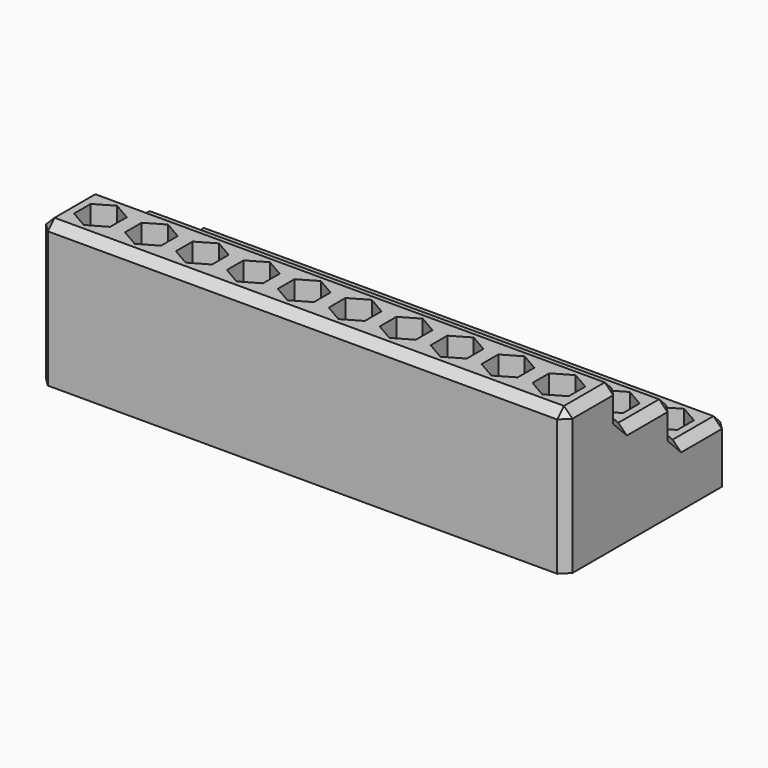
from build123d import *

# Parameters (mm, degrees)
F2_W     = 62
F2_H     = 8
F3_DEPTH = 17
F4_DEPTH = 12
F5_DEPTH = 7
F6_DEPTH = 8
F7_DEPTH = 13
F8_DEPTH = 18
F9_SIZE  = 1


with BuildPart() as f3:
    # F2 (on offset) → F3 (new body)
    with BuildSketch(Plane.XY.offset(-20)):
        with Locations((31, 4)):
            Rectangle(F2_W, F2_H)
    extrude(amount=F3_DEPTH)

    # F2 (on offset) → F4 (join)
    with BuildSketch(Plane.XY.offset(-20)):
        with Locations((31, 12)):
            Rectangle(F2_W, F2_H)
    extrude(amount=F4_DEPTH)

    # F2 (on offset) → F5 (join)
    with BuildSketch(Plane.XY.offset(-20)):
        with Locations((31, 20)):
            Rectangle(F2_W, F2_H)
    extrude(amount=F5_DEPTH)

    # F0 (on Top) → F6 (cut)
    with BuildSketch(Plane.XY):
        Polygon((58, 6.4537386441), (55.875, 5.226869322), (55.875, 2.773130678), (58, 1.5462613559), (60.125, 2.773130678), (60.125, 5.226869322), align=None)
        Polygon((52, 6.4537386441), (49.875, 5.226869322), (49.875, 2.773130678), (52, 1.5462613559), (54.125, 2.773130678), (54.125, 5.226869322), align=None)
        Polygon((46, 6.4537386441), (43.875, 5.226869322), (43.875, 2.773130678), (46, 1.5462613559), (48.125, 2.773130678), (48.125, 5.226869322), align=None)
        Polygon((40, 6.4537386441), (37.875, 5.226869322), (37.875, 2.773130678), (40, 1.5462613559), (42.125, 2.773130678), (42.125, 5.226869322), align=None)
        Polygon((34, 6.4537386441), (31.875, 5.226869322), (31.875, 2.773130678), (34, 1.5462613559), (36.125, 2.773130678), (36.125, 5.226869322), align=None)
        Polygon((28, 6.4537386441), (25.875, 5.226869322), (25.875, 2.773130678), (28, 1.5462613559), (30.125, 2.773130678), (30.125, 5.226869322), align=None)
        Polygon((22, 6.4537386441), (19.875, 5.226869322), (19.875, 2.773130678), (22, 1.5462613559), (24.125, 2.773130678), (24.125, 5.226869322), align=None)
        Polygon((16, 6.4537386441), (13.875, 5.226869322), (13.875, 2.773130678), (16, 1.5462613559), (18.125, 2.773130678), (18.125, 5.226869322), align=None)
        Polygon((10, 6.4537386441), (7.875, 5.226869322), (7.875, 2.773130678), (10, 1.5462613559), (12.125, 2.773130678), (12.125, 5.226869322), align=None)
        Polygon((1.875, 5.226869322), (1.875, 2.773130678), (4, 1.5462613559), (6.125, 2.773130678), (6.125, 5.226869322), (4, 6.4537386441), align=None)
    extrude(amount=-F6_DEPTH, mode=Mode.SUBTRACT)

    # F0 (on Top) → F7 (cut)
    with BuildSketch(Plane.XY):
        Polygon((58, 14.4537386441), (55.875, 13.226869322), (55.875, 10.773130678), (58, 9.5462613559), (60.125, 10.773130678), (60.125, 13.226869322), align=None)
        Polygon((52, 14.4537386441), (49.875, 13.226869322), (49.875, 10.773130678), (52, 9.5462613559), (54.125, 10.773130678), (54.125, 13.226869322), align=None)
        Polygon((43.875, 10.773130678), (46, 9.5462613559), (48.125, 10.773130678), (48.125, 13.226869322), (46, 14.4537386441), (43.875, 13.226869322), align=None)
        Polygon((37.875, 10.773130678), (40, 9.5462613559), (42.125, 10.773130678), (42.125, 13.226869322), (40, 14.4537386441), (37.875, 13.226869322), align=None)
        Polygon((36.125, 10.773130678), (36.125, 13.226869322), (34, 14.4537386441), (31.875, 13.226869322), (31.875, 10.773130678), (34, 9.5462613559), align=None)
        Polygon((30.125, 10.773130678), (30.125, 13.226869322), (28, 14.4537386441), (25.875, 13.226869322), (25.875, 10.773130678), (28, 9.5462613559), align=None)
        Polygon((22, 14.4537386441), (19.875, 13.226869322), (19.875, 10.773130678), (22, 9.5462613559), (24.125, 10.773130678), (24.125, 13.226869322), align=None)
        Polygon((16, 14.4537386441), (13.875, 13.226869322), (13.875, 10.773130678), (16, 9.5462613559), (18.125, 10.773130678), (18.125, 13.226869322), align=None)
        Polygon((12.125, 13.226869322), (10, 14.4537386441), (7.875, 13.226869322), (7.875, 10.773130678), (10, 9.5462613559), (12.125, 10.773130678), align=None)
        Polygon((4, 14.4537386441), (1.875, 13.226869322), (1.875, 10.773130678), (4, 9.5462613559), (6.125, 10.773130678), (6.125, 13.226869322), align=None)
    extrude(amount=-F7_DEPTH, mode=Mode.SUBTRACT)

    # F0 (on Top) → F8 (cut)
    with BuildSketch(Plane.XY):
        Polygon((58, 22.4537386441), (55.875, 21.226869322), (55.875, 18.773130678), (58, 17.5462613559), (60.125, 18.773130678), (60.125, 21.226869322), align=None)
        Polygon((52, 22.4537386441), (49.875, 21.226869322), (49.875, 18.773130678), (52, 17.5462613559), (54.125, 18.773130678), (54.125, 21.226869322), align=None)
        Polygon((43.875, 18.773130678), (46, 17.5462613559), (48.125, 18.773130678), (48.125, 21.226869322), (46, 22.4537386441), (43.875, 21.226869322), align=None)
        Polygon((37.875, 18.773130678), (40, 17.5462613559), (42.125, 18.773130678), (42.125, 21.226869322), (40, 22.4537386441), (37.875, 21.226869322), align=None)
        Polygon((36.125, 18.773130678), (36.125, 21.226869322), (34, 22.4537386441), (31.875, 21.226869322), (31.875, 18.773130678), (34, 17.5462613559), align=None)
        Polygon((30.125, 18.773130678), (30.125, 21.226869322), (28, 22.4537386441), (25.875, 21.226869322), (25.875, 18.773130678), (28, 17.5462613559), align=None)
        Polygon((22, 22.4537386441), (19.875, 21.226869322), (19.875, 18.773130678), (22, 17.5462613559), (24.125, 18.773130678), (24.125, 21.226869322), align=None)
        Polygon((16, 22.4537386441), (13.875, 21.226869322), (13.875, 18.773130678), (16, 17.5462613559), (18.125, 18.773130678), (18.125, 21.226869322), align=None)
        Polygon((12.125, 21.226869322), (10, 22.4537386441), (7.875, 21.226869322), (7.875, 18.773130678), (10, 17.5462613559), (12.125, 18.773130678), align=None)
        Polygon((4, 22.4537386441), (1.875, 21.226869322), (1.875, 18.773130678), (4, 17.5462613559), (6.125, 18.773130678), (6.125, 21.226869322), align=None)
    extrude(amount=-F8_DEPTH, mode=Mode.SUBTRACT)

    # F9
    f9_edges = [f3.edges().sort_by_distance(p)[0] for p in [
        (31, 8, -3),
        (31, 16, -8),
        (31, 24, -13),
        (31, 16, -13),
        (31, 8, -8),
        (62, 4, -3),
        (62, 12, -8),
        (62, 20, -13),
        (31, 0, -3),
        (62, 0, -11.5),
        (62, 24, -16.5),
        (0, 24, -16.5),
        (0, 20, -13),
        (0, 12, -8),
        (0, 4, -3),
        (0, 0, -11.5),
        (0, 8, -5.5),
        (62, 8, -5.5),
        (0, 16, -10.5),
        (62, 16, -10.5),
    ]]
    chamfer(f9_edges, length=F9_SIZE)


solid = f3.part
